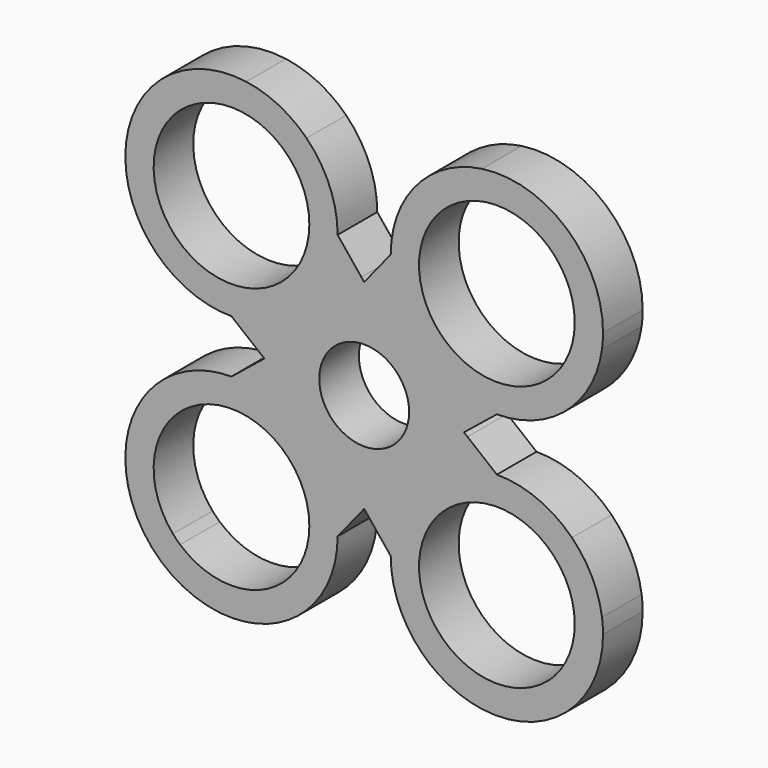
from build123d import *
from build123d import SkipClean  # not in build123d's __all__

# Parameters (mm, degrees)
F0_R     = 37.5
F1_DEPTH = 7
F2_R     = 6.35
F3_DEPTH = 7.001
F5_DEPTH = 7.001
F7_DEPTH = 7
F9_DEPTH = 7.001


with BuildPart() as f1:
    # F0 (on Front) → F1 (new body)
    with BuildSketch(Plane.XZ):
        Circle(F0_R)
    extrude(amount=F1_DEPTH)

    # F2 (on face) → F3 (cut, through all)
    with BuildSketch(Plane.XZ.offset(7)):
        Circle(F2_R)
    extrude(amount=-F3_DEPTH, mode=Mode.SUBTRACT)

    # F4 (on face) → F5 (cut, through all)
    with BuildSketch(Plane.XZ.offset(7)):
        with BuildLine():
            Line((-8.1433982822, 29.3566017178), (0, 37.5))
            ThreePointArc((0, 37.5), (-8.5491327229, 36.5124955281), (-16.6480090834, 33.6019909166))
            ThreePointArc((-16.6480090834, 33.6019909166), (-12.0505288232, 32.1707706914), (-8.1433982822, 29.3566017178))
        make_face()
        with BuildLine():
            ThreePointArc((16.6480090834, 33.6019909166), (8.5491327229, 36.5124955281), (0, 37.5))
            Line((0, 37.5), (8.1433982822, 29.3566017178))
            ThreePointArc((8.1433982822, 29.3566017178), (12.0505288232, 32.1707706914), (16.6480090834, 33.6019909166))
        make_face()
        with BuildLine():
            Line((0, 18.75), (0, 37.5))
            Line((0, 37.5), (-8.1433982822, 29.3566017178))
            ThreePointArc((-8.1433982822, 29.3566017178), (-4.8918070123, 24.4902514855), (-3.75, 18.75))
            Line((-3.75, 18.75), (0, 18.75))
        make_face()
        with BuildLine():
            Line((8.1433982822, 29.3566017178), (0, 37.5))
            Line((0, 37.5), (0, 18.75))
            Line((0, 18.75), (3.75, 18.75))
            ThreePointArc((3.75, 18.75), (4.8918070123, 24.4902514855), (8.1433982822, 29.3566017178))
        make_face()
        Polygon((0, 15), (0, 18.75), (-3.75, 18.75), align=None)
        Polygon((0, 15), (-3.75, 18.75), (-0.4017027864, 14.5982972136), align=None)
        Polygon((3.75, 18.75), (0, 18.75), (0, 15), align=None)
        Polygon((0.4017027864, 14.5982972136), (3.75, 18.75), (0, 15), align=None)
        with BuildLine():
            Line((-29.3566017178, -8.1433982822), (-37.5, 0))
            ThreePointArc((-37.5, 0), (-36.5124955281, -8.5491327229), (-33.6019909166, -16.6480090834))
            ThreePointArc((-33.6019909166, -16.6480090834), (-32.1707706914, -12.0505288232), (-29.3566017178, -8.1433982822))
        make_face()
        with BuildLine():
            ThreePointArc((-29.3566017178, 8.1433982822), (-32.1707706914, 12.0505288232), (-33.6019909166, 16.6480090834))
            ThreePointArc((-33.6019909166, 16.6480090834), (-36.5124955281, 8.5491327229), (-37.5, 0))
            Line((-37.5, 0), (-29.3566017178, 8.1433982822))
        make_face()
        with BuildLine():
            ThreePointArc((-18.75, 3.75), (-24.4902514855, 4.8918070123), (-29.3566017178, 8.1433982822))
            Line((-29.3566017178, 8.1433982822), (-37.5, 0))
            Line((-37.5, 0), (-18.75, 0))
            Line((-18.75, 0), (-18.75, 3.75))
        make_face()
        with BuildLine():
            Line((-18.75, 0), (-37.5, 0))
            Line((-37.5, 0), (-29.3566017178, -8.1433982822))
            ThreePointArc((-29.3566017178, -8.1433982822), (-24.4902514855, -4.8918070123), (-18.75, -3.75))
            Line((-18.75, -3.75), (-18.75, 0))
        make_face()
        Polygon((0.4017027864, 14.5982972136), (0, 15), (0, 14.1002080444), align=None)
        Polygon((0, 14.1002080444), (0, 15), (-0.4017027864, 14.5982972136), align=None)
        Polygon((-15, 0), (-18.75, 3.75), (-18.75, 0), align=None)
        Polygon((-14.5982972136, 0.4017027864), (-18.75, 3.75), (-15, 0), align=None)
        Polygon((-14.5982972136, 0.4017027864), (-15, 0), (-14.1002080444, 0), align=None)
        Polygon((-14.1002080444, 0), (-15, 0), (-14.5982972136, -0.4017027864), align=None)
        Polygon((-14.5982972136, -0.4017027864), (-15, 0), (-18.75, -3.75), align=None)
        Polygon((-15, 0), (-18.75, 0), (-18.75, -3.75), align=None)
        with BuildLine():
            ThreePointArc((-8.1433982822, -29.3566017178), (-12.0505288232, -32.1707706914), (-16.6480090834, -33.6019909166))
            ThreePointArc((-16.6480090834, -33.6019909166), (-8.5491327229, -36.5124955281), (0, -37.5))
            Line((0, -37.5), (-8.1433982822, -29.3566017178))
        make_face()
        with BuildLine():
            ThreePointArc((0, -37.5), (8.5491327229, -36.5124955281), (16.6480090834, -33.6019909166))
            ThreePointArc((16.6480090834, -33.6019909166), (12.0505288232, -32.1707706914), (8.1433982822, -29.3566017178))
            Line((8.1433982822, -29.3566017178), (0, -37.5))
        make_face()
        with BuildLine():
            Line((0, -37.5), (8.1433982822, -29.3566017178))
            ThreePointArc((8.1433982822, -29.3566017178), (4.8918070123, -24.4902514855), (3.75, -18.75))
            Line((3.75, -18.75), (0, -18.75))
            Line((0, -18.75), (0, -37.5))
        make_face()
        with BuildLine():
            Line((-8.1433982822, -29.3566017178), (0, -37.5))
            Line((0, -37.5), (0, -18.75))
            Line((0, -18.75), (-3.75, -18.75))
            ThreePointArc((-3.75, -18.75), (-4.8918070123, -24.4902514855), (-8.1433982822, -29.3566017178))
        make_face()
        Polygon((-0.4017027864, -14.5982972136), (0, -15), (0, -14.1002080444), align=None)
        Polygon((0, -14.1002080444), (0, -15), (0.4017027864, -14.5982972136), align=None)
        Polygon((0, -15), (3.75, -18.75), (0.4017027864, -14.5982972136), align=None)
        Polygon((-0.4017027864, -14.5982972136), (-3.75, -18.75), (0, -15), align=None)
        Polygon((0, -15), (-3.75, -18.75), (0, -18.75), align=None)
        Polygon((0, -18.75), (3.75, -18.75), (0, -15), align=None)
        with BuildLine():
            ThreePointArc((37.5, 0), (36.5124955281, 8.5491327229), (33.6019909166, 16.6480090834))
            ThreePointArc((33.6019909166, 16.6480090834), (32.1707706914, 12.0505288232), (29.3566017178, 8.1433982822))
            Line((29.3566017178, 8.1433982822), (37.5, 0))
        make_face()
        with BuildLine():
            Line((37.5, 0), (29.3566017178, 8.1433982822))
            ThreePointArc((29.3566017178, 8.1433982822), (24.4902514855, 4.8918070123), (18.75, 3.75))
            Line((18.75, 3.75), (18.75, 0))
            Line((18.75, 0), (37.5, 0))
        make_face()
        with BuildLine():
            ThreePointArc((33.6019909166, -16.6480090834), (36.5124955281, -8.5491327229), (37.5, 0))
            Line((37.5, 0), (29.3566017178, -8.1433982822))
            ThreePointArc((29.3566017178, -8.1433982822), (32.1707706914, -12.0505288232), (33.6019909166, -16.6480090834))
        make_face()
        with BuildLine():
            Line((29.3566017178, -8.1433982822), (37.5, 0))
            Line((37.5, 0), (18.75, 0))
            Line((18.75, 0), (18.75, -3.75))
            ThreePointArc((18.75, -3.75), (24.4902514855, -4.8918070123), (29.3566017178, -8.1433982822))
        make_face()
        Polygon((15, 0), (18.75, 3.75), (14.5982972136, 0.4017027864), align=None)
        Polygon((18.75, 0), (18.75, 3.75), (15, 0), align=None)
        Polygon((18.75, -3.75), (18.75, 0), (15, 0), align=None)
        Polygon((18.75, -3.75), (15, 0), (14.5982972136, -0.4017027864), align=None)
        Polygon((14.5982972136, -0.4017027864), (15, 0), (14.1002080444, 0), align=None)
        Polygon((14.1002080444, 0), (15, 0), (14.5982972136, 0.4017027864), align=None)
    extrude(amount=-F5_DEPTH, mode=Mode.SUBTRACT)

    # F6 (on face) → F7 (join)
    with BuildSketch(Plane.XZ.offset(7)):
        with BuildLine():
            ThreePointArc((-33.6019909166, 16.6480090834), (-26.5165042945, 26.5165042945), (-16.6480090834, 33.6019909166))
            ThreePointArc((-16.6480090834, 33.6019909166), (-29.3566017178, 29.3566017178), (-33.6019909166, 16.6480090834))
        make_face()
        with BuildLine():
            ThreePointArc((-16.6480090834, -33.6019909166), (-26.5165042945, -26.5165042945), (-33.6019909166, -16.6480090834))
            ThreePointArc((-33.6019909166, -16.6480090834), (-29.3566017178, -29.3566017178), (-16.6480090834, -33.6019909166))
        make_face()
        with BuildLine():
            ThreePointArc((33.75, -18.75), (33.7129519773, -17.6964022943), (33.6019909166, -16.6480090834))
            ThreePointArc((33.6019909166, -16.6480090834), (26.5165042945, -26.5165042945), (16.6480090834, -33.6019909166))
            ThreePointArc((16.6480090834, -33.6019909166), (28.5853987273, -30.0754108921), (33.75, -18.75))
        make_face()
        with BuildLine():
            ThreePointArc((33.75, 18.75), (28.5853987273, 30.0754108921), (16.6480090834, 33.6019909166))
            ThreePointArc((16.6480090834, 33.6019909166), (26.5165042945, 26.5165042945), (33.6019909166, 16.6480090834))
            ThreePointArc((33.6019909166, 16.6480090834), (33.7129519773, 17.6964022943), (33.75, 18.75))
        make_face()
    with SkipClean():  # cleaning this boolean's faces spoils the solid; the shape is the same uncleaned
        extrude(amount=-F7_DEPTH)

    # F8 (on face) → F9 (cut, through all)
    with BuildSketch(Plane.XZ.offset(7)):
        with BuildLine():
            ThreePointArc((-27.0181551222, 26.0051782112), (-26.5165042945, 26.5165042945), (-26.0051782112, 27.0181551222))
            ThreePointArc((-26.0051782112, 27.0181551222), (-26.5281745931, 26.5281745931), (-27.0181551222, 26.0051782112))
        make_face()
        with BuildLine():
            ThreePointArc((-27.0181551222, 26.0051782112), (-22.6262284283, 8.4555911694), (-7.75, 18.75))
            ThreePointArc((-7.75, 18.75), (-14.2116611146, 28.7701536995), (-26.0051782112, 27.0181551222))
            ThreePointArc((-26.0051782112, 27.0181551222), (-26.5165042945, 26.5165042945), (-27.0181551222, 26.0051782112))
        make_face()
        with BuildLine():
            ThreePointArc((27.0181551222, 26.0051782112), (26.5281745931, 26.5281745931), (26.0051782112, 27.0181551222))
            ThreePointArc((26.0051782112, 27.0181551222), (26.5165042945, 26.5165042945), (27.0181551222, 26.0051782112))
        make_face()
        with BuildLine():
            ThreePointArc((27.0181551222, 26.0051782112), (26.5165042945, 26.5165042945), (26.0051782112, 27.0181551222))
            ThreePointArc((26.0051782112, 27.0181551222), (8.7298463005, 14.2116611146), (29.75, 18.75))
            ThreePointArc((29.75, 18.75), (29.0444088306, 22.6262284283), (27.0181551222, 26.0051782112))
        make_face()
        with BuildLine():
            ThreePointArc((26.0051782112, -27.0181551222), (26.5281745931, -26.5281745931), (27.0181551222, -26.0051782112))
            ThreePointArc((27.0181551222, -26.0051782112), (26.5165042945, -26.5165042945), (26.0051782112, -27.0181551222))
        make_face()
        with BuildLine():
            ThreePointArc((26.0051782112, -27.0181551222), (26.5165042945, -26.5165042945), (27.0181551222, -26.0051782112))
            ThreePointArc((27.0181551222, -26.0051782112), (29.0444088306, -22.6262284283), (29.75, -18.75))
            ThreePointArc((29.75, -18.75), (8.7298463005, -14.2116611146), (26.0051782112, -27.0181551222))
        make_face()
        with BuildLine():
            ThreePointArc((-26.0051782112, -27.0181551222), (-26.5165042945, -26.5165042945), (-27.0181551222, -26.0051782112))
            ThreePointArc((-27.0181551222, -26.0051782112), (-26.5281745931, -26.5281745931), (-26.0051782112, -27.0181551222))
        make_face()
        with BuildLine():
            ThreePointArc((-7.75, -18.75), (-22.6262284283, -8.4555911694), (-27.0181551222, -26.0051782112))
            ThreePointArc((-27.0181551222, -26.0051782112), (-26.5165042945, -26.5165042945), (-26.0051782112, -27.0181551222))
            ThreePointArc((-26.0051782112, -27.0181551222), (-14.2116611146, -28.7701536995), (-7.75, -18.75))
        make_face()
    extrude(amount=-F9_DEPTH, mode=Mode.SUBTRACT)


solid = f1.part
